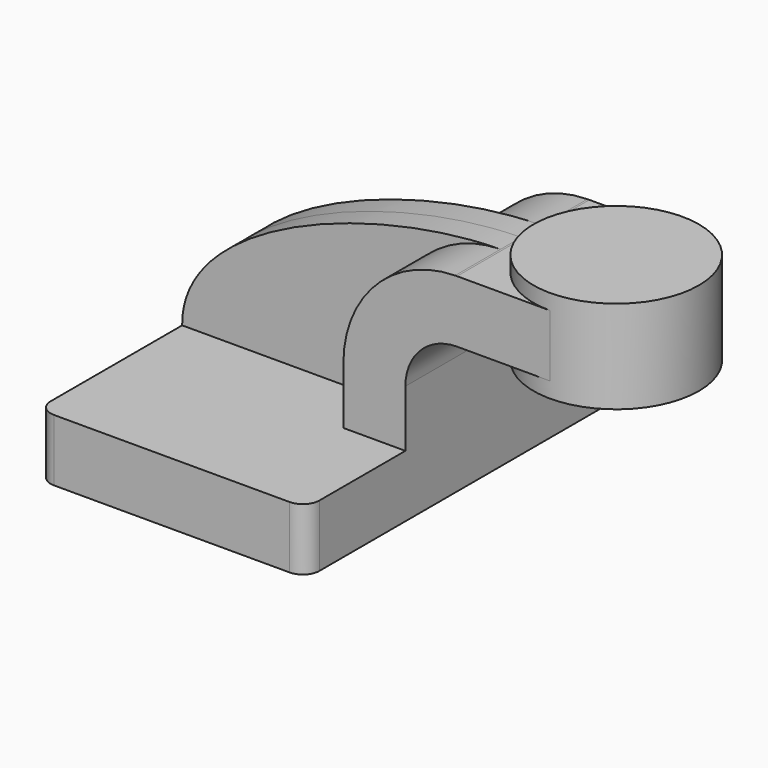
from build123d import *

# Parameters (mm, degrees)
F1_DEPTH = 63.5
F2_DEPTH = 7.9375
F3_DEPTH = 25.4
F0_W     = 25.4
F0_H     = 19.05
F4_DEPTH = 25.4
F6_R     = 5.08


# Not quite as in the source:
# - a feature names something its author has since deleted; it is built from what else it names


with BuildPart() as f1:
    # F0 (on Front) → F1 (new body, symmetric)
    with BuildSketch(Plane.XZ):
        Polygon((22.225, 9.525), (-41.275, 9.525), (-41.275, -9.525), (41.275, -9.525), (41.275, 9.525), align=None)
    extrude(amount=F1_DEPTH, both=True)

    # F0 (on Front) → F2 (join, symmetric)
    with BuildSketch(Plane.XZ):
        with BuildLine():
            add(Edge.make_bspline(
                [(-41.275, 9.525), (-41.6611139955, 40.1644010986), (17.1509007839, 61.4882749154), (56.5663251016, 61.9203224026)],
                knots=[0, 0, 0, 0, 110.9555033405, 110.9555033405, 110.9555033405, 110.9555033405], degree=3))
            Line((-41.275, 9.525), (22.225, 9.525))
            Line((22.225, 9.525), (22.225, 27.0002))
            ThreePointArc((22.225, 27.0002), (32.2487904829, 51.4886746276), (56.5663251016, 61.9203224026))
        make_face()
    extrude(amount=F2_DEPTH, both=True)

    # F0 (on Front) → F3 (join, symmetric)
    with BuildSketch(Plane.XZ):
        with BuildLine():
            Line((22.225, 27.0002), (22.225, 9.525))
            Line((22.225, 9.525), (41.275, 9.525))
            Line((41.275, 9.525), (41.275, 27.0002))
            ThreePointArc((41.275, 27.0002), (45.9246798487, 38.2255201513), (57.15, 42.8752))
            Line((57.15, 42.8752), (60.325, 42.8752))
            Line((60.325, 42.8752), (60.325, 61.9252))
            Line((60.325, 61.9252), (57.15, 61.9252))
            add(Edge.make_bspline(
                [(56.5663251016, 61.9203224026), (56.7613614994, 61.9224602709), (56.955922973, 61.9240866042), (57.15, 61.9252)],
                knots=[110.9555033405, 110.9555033405, 110.9555033405, 110.9555033405, 111.5045361635, 111.5045361635, 111.5045361635, 111.5045361635], degree=3))
            ThreePointArc((56.5663251016, 61.9203224026), (32.2487904829, 51.4886746276), (22.225, 27.0002))
        make_face()
    extrude(amount=F3_DEPTH, both=True)

    # F0 (on Front) → F4 (join, symmetric)
    with BuildSketch(Plane.XZ):
        with Locations((73.025, 52.4002)):
            Rectangle(F0_W, F0_H)
    extrude(amount=F4_DEPTH, both=True)

    # F0 (on Front) → F5 (revolve)
    with BuildSketch(Plane.XZ):
        Polygon((85.725, 66.675), (85.725, 61.9252), (85.725, 42.8752), (85.725, 38.1), (111.125, 38.1), (111.125, 66.675), align=None)
    revolve(axis=Axis((85.725, 0, 52.3875), (0, 0, 1)))

    # F6
    f6_edges = [f1.edges().sort_by_distance(p)[0] for p in [
        (-41.275, -63.5, 0),
        (41.275, -63.5, 0),
        (41.275, 63.5, 0),
        (-41.275, 63.5, 0),
    ]]
    fillet(f6_edges, radius=F6_R)


solid = f1.part
